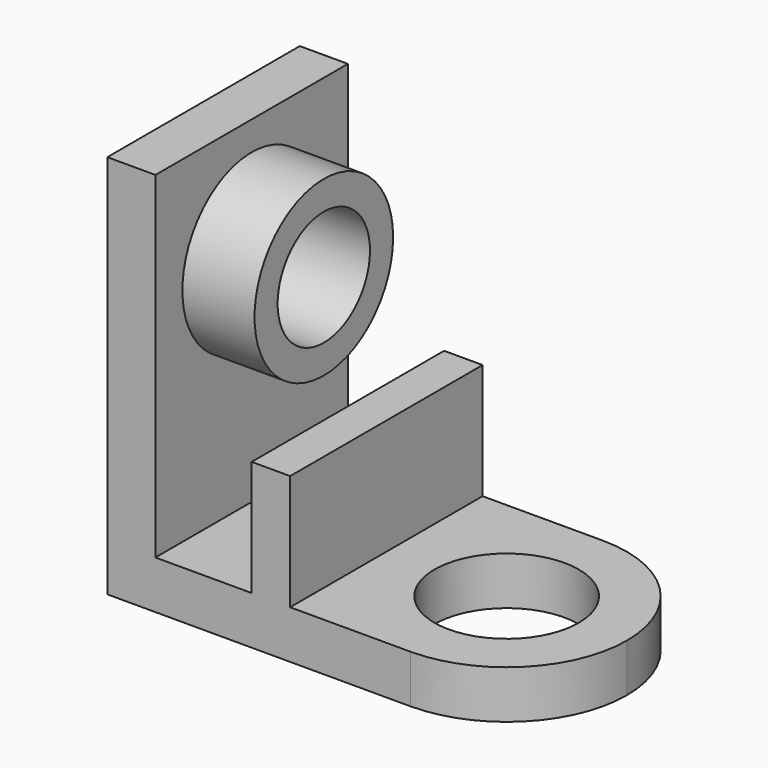
from build123d import *

# Parameters (mm, degrees)
F1_DEPTH = 50
F2_R     = 25
F3_R     = 24.99999
F4_R     = 15
F5_DEPTH = 10
F6_R     = 18
F7_DEPTH = 15
F8_R     = 12
F9_DEPTH = 25


# Not quite as in the source:
# - a fillet or chamfer is up to 0.001 mm smaller than in the source, because OpenCascade refuses the exact size


with BuildPart() as f1:
    # F0 (on Front) → F1 (new body)
    with BuildSketch(Plane.XZ):
        Polygon((0, 80), (0, 0), (88, 0), (88, 10), (38, 10), (38, 34), (30, 34), (30, 10), (10, 10), (10, 80), align=None)
    extrude(amount=F1_DEPTH)

    # F2
    f2_edges = [f1.edges().sort_by_distance(p)[0] for p in [
        (88, -50, 5),
    ]]
    fillet(f2_edges, radius=F2_R)

    # F3 (radius 25 in the source; OpenCascade refuses exactly that, so slightly less here)
    f3_edges = [f1.edges().sort_by_distance(p)[0] for p in [
        (88, 0, 5),
    ]]
    fillet(f3_edges, radius=F3_R)

    # F4 (on face) → F5 (cut, through all)
    with BuildSketch(Plane.XY.offset(10)):
        with Locations((63, -25)):
            Circle(F4_R)
    extrude(amount=-F5_DEPTH, mode=Mode.SUBTRACT)

    # F6 (on face) → F7 (join)
    with BuildSketch(Plane.YZ.offset(10)):
        with Locations((-25, 56)):
            Circle(F6_R)
    extrude(amount=F7_DEPTH)

    # F8 (on face) → F9 (cut, through all)
    with BuildSketch(Plane.YZ.offset(25)):
        with Locations((-25, 56)):
            Circle(F8_R)
    extrude(amount=-F9_DEPTH, mode=Mode.SUBTRACT)


solid = f1.part
